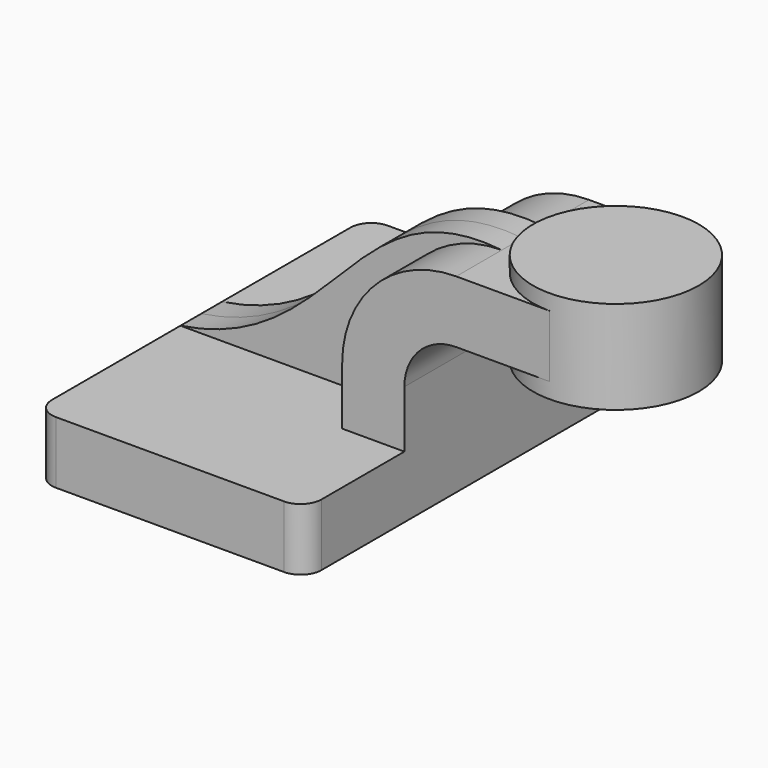
from build123d import *

# Parameters (mm, degrees)
F1_DEPTH = 63.5
F0_W     = 25.4
F0_H     = 19.05
F2_DEPTH = 25.4
F3_DEPTH = 7.9375
F5_R     = 6.35


# Not quite as in the source:
# - a feature names something its author has since deleted; it is built from what else it names


with BuildPart() as f1:
    # F0 (on Front) → F1 (new body, symmetric)
    with BuildSketch(Plane.XZ):
        Polygon((41.275, -9.525), (41.275, 9.525), (22.225, 9.525), (-41.275, 9.525), (-41.275, -9.525), align=None)
    extrude(amount=F1_DEPTH, both=True)

    # F0 (on Front) → F2 (join, symmetric)
    with BuildSketch(Plane.XZ):
        with BuildLine():
            Line((22.225, 9.525), (41.275, 9.525))
            Line((41.275, 9.525), (41.275, 27.0002))
            ThreePointArc((41.275, 27.0002), (45.9246798487, 38.2255201513), (57.15, 42.8752))
            Line((57.15, 42.8752), (60.325, 42.8752))
            Line((60.325, 42.8752), (60.325, 61.9252))
            Line((60.325, 61.9252), (57.15, 61.9252))
            ThreePointArc((57.15, 61.9252), (32.4542956671, 51.6959043329), (22.225, 27.0002))
            Line((22.225, 27.0002), (22.225, 9.525))
        make_face()
        with Locations((73.025, 52.4002)):
            Rectangle(F0_W, F0_H)
    extrude(amount=F2_DEPTH, both=True)

    # F0 (on Front) → F3 (join, symmetric)
    with BuildSketch(Plane.XZ):
        with BuildLine():
            Line((-41.275, 9.525), (22.225, 9.525))
            Line((22.225, 9.525), (22.225, 27.0002))
            ThreePointArc((22.225, 27.0002), (32.4542956671, 51.6959043329), (57.15, 61.9252))
            add(Edge.make_bspline(
                [(-41.275, 9.525), (7.2152586654, 16.9252250344), (10.756178759, 66.7510330677), (57.15, 61.9252)],
                knots=[0, 0, 0, 0, 111.5045361635, 111.5045361635, 111.5045361635, 111.5045361635], degree=3))
        make_face()
    extrude(amount=F3_DEPTH, both=True)

    # F0 (on Front) → F4 (revolve)
    with BuildSketch(Plane.XZ):
        Polygon((85.725, 61.9252), (85.725, 42.8752), (85.725, 38.1), (111.125, 38.1), (111.125, 66.675), (85.725, 66.675), align=None)
    revolve(axis=Axis((85.725, 0, 52.3875), (0, 0, -1)))

    # F5
    f5_edges = [f1.edges().sort_by_distance(p)[0] for p in [
        (41.275, -63.5, 0),
        (-41.275, -63.5, 0),
        (41.275, 63.5, 0),
        (-41.275, 63.5, 0),
    ]]
    fillet(f5_edges, radius=F5_R)


solid = f1.part
